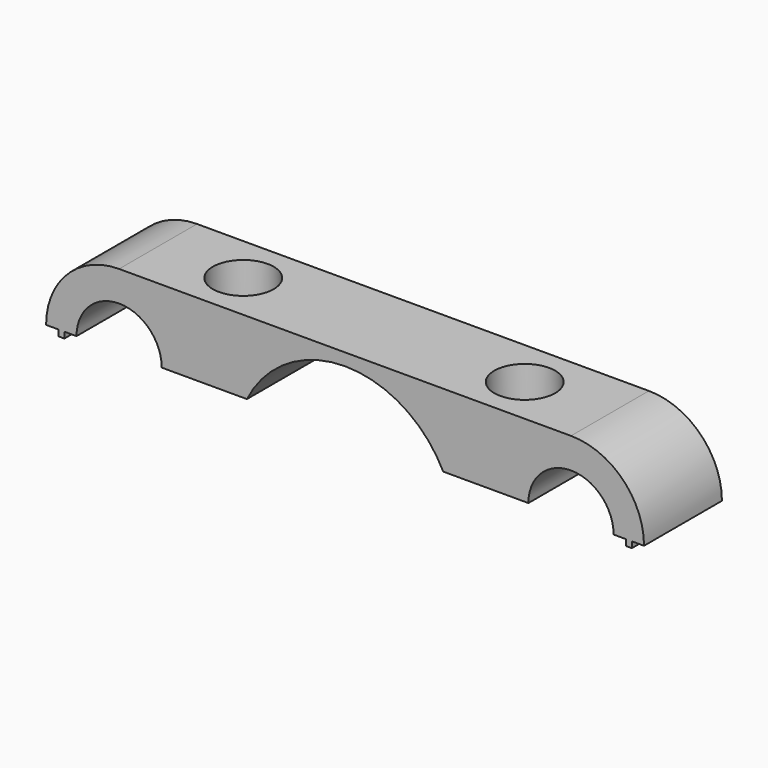
from build123d import *

# Parameters (mm, degrees)
F1_DEPTH       = 8
F3_D           = 5
F3_CBORE_D     = 10
F3_CBORE_DEPTH = 6
F4_R           = 11.99999
F5_W           = 1
F5_H           = 16
F6_DEPTH       = 1
F7_W           = 1
F7_H           = 16
F8_DEPTH       = 1


# Not quite as in the source:
# - a fillet or chamfer is up to 0.001 mm smaller than in the source, because OpenCascade refuses the exact size
# - a feature names something its author has since deleted; it is built from what else it names


with BuildPart() as f1:
    # F0 (on Front) → F1 (new body, symmetric)
    with BuildSketch(Plane.XZ):
        with BuildLine():
            Line((-49.125, -6), (-44.125, -6))
            ThreePointArc((-44.125, -6), (-37.125, 1), (-30.125, -6))
            Line((-30.125, -6), (-16.1245154966, -6))
            ThreePointArc((-16.1245154966, -6), (0, 4), (16.1245154966, -6))
            Line((16.1245154966, -6), (30.125, -6))
            ThreePointArc((30.125, -6), (37.125, 1), (44.125, -6))
            Line((44.125, -6), (49.125, -6))
            Line((49.125, -6), (49.125, 6))
            Line((49.125, 6), (-49.125, 6))
            Line((-49.125, 6), (-49.125, -6))
        make_face()
    extrude(amount=F1_DEPTH, both=True)

    # F3 (through all)
    with Locations(Plane.XY.offset(6)):
        with Locations((-23.125, 0), (23.125, 0)):
            CounterBoreHole(F3_D / 2, F3_CBORE_D / 2, F3_CBORE_DEPTH)

    # F4 (radius 12 in the source; OpenCascade refuses exactly that, so slightly less here)
    f4_edges = [f1.edges().sort_by_distance(p)[0] for p in [
        (49.125, 0, 6),
        (-49.125, 0, 6),
    ]]
    fillet(f4_edges, radius=F4_R)

    # F5 (on face) → F6 (join)
    with BuildSketch(Plane(origin=(0, 0, -6), x_dir=(1, 0, 0), z_dir=(0, 0, -1))):
        with Locations((-46.625, 0)):
            Rectangle(F5_W, F5_H)
    extrude(amount=F6_DEPTH)

    # F7 (on face) → F8 (join)
    with BuildSketch(Plane(origin=(0, 0, -6), x_dir=(1, 0, 0), z_dir=(0, 0, -1))):
        with Locations((46.625, 0)):
            Rectangle(F7_W, F7_H)
    extrude(amount=F8_DEPTH)


solid = f1.part
